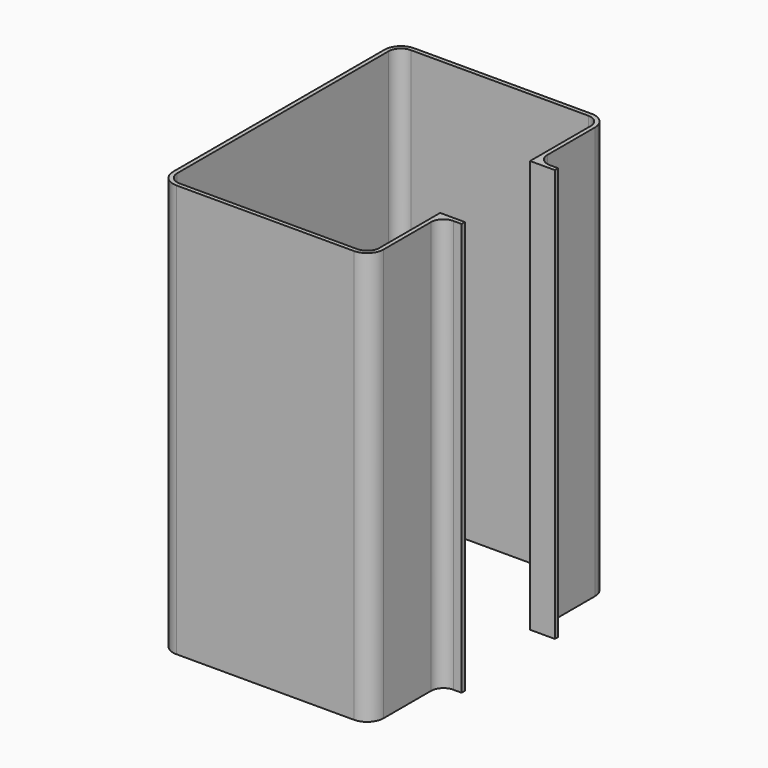
from build123d import *

# Parameters (mm, degrees)
F1_DEPTH = 100


# Not quite as in the source:
# - a feature names something its author has since deleted; it is built from what else it names


with BuildPart() as f1:
    # F0 (on Top) → F1 (new body)
    with BuildSketch(Plane.XY):
        with BuildLine():
            Line((-21.5, 35), (21.5, 35))
            ThreePointArc((21.5, 35), (23.6213203436, 34.1213203436), (24.5, 32))
            Line((24.5, 32), (24.5, 13.625))
            Line((24.5, 13.625), (30.5, 13.625))
            Line((30.5, 13.625), (30.5, 14.625))
            Line((30.5, 14.625), (28.5, 14.625))
            ThreePointArc((28.5, 14.625), (26.3786796564, 15.5036796564), (25.5, 17.625))
            Line((25.5, 17.625), (25.5, 32))
            ThreePointArc((25.5, 32), (24.3284271247, 34.8284271247), (21.5, 36))
            Line((21.5, 36), (-21.5, 36))
            ThreePointArc((-21.5, 36), (-24.3284271247, 34.8284271247), (-25.5, 32))
            Line((-25.5, 32), (-25.5, -32))
            ThreePointArc((-25.5, -32), (-24.3284271247, -34.8284271247), (-21.5, -36))
            Line((-21.5, -36), (21.5, -36))
            ThreePointArc((21.5, -36), (24.3284271247, -34.8284271247), (25.5, -32))
            Line((25.5, -32), (25.5, -17.625))
            ThreePointArc((25.5, -17.625), (26.3786796564, -15.5036796564), (28.5, -14.625))
            Line((28.5, -14.625), (30.5, -14.625))
            Line((30.5, -14.625), (30.5, -13.625))
            Line((30.5, -13.625), (24.5, -13.625))
            Line((24.5, -13.625), (24.5, -32))
            ThreePointArc((24.5, -32), (23.6213203436, -34.1213203436), (21.5, -35))
            Line((21.5, -35), (-21.5, -35))
            ThreePointArc((-21.5, -35), (-23.6213203436, -34.1213203436), (-24.5, -32))
            Line((-24.5, -32), (-24.5, 32))
            ThreePointArc((-24.5, 32), (-23.6213203436, 34.1213203436), (-21.5, 35))
        make_face()
    extrude(amount=F1_DEPTH)


solid = f1.part
